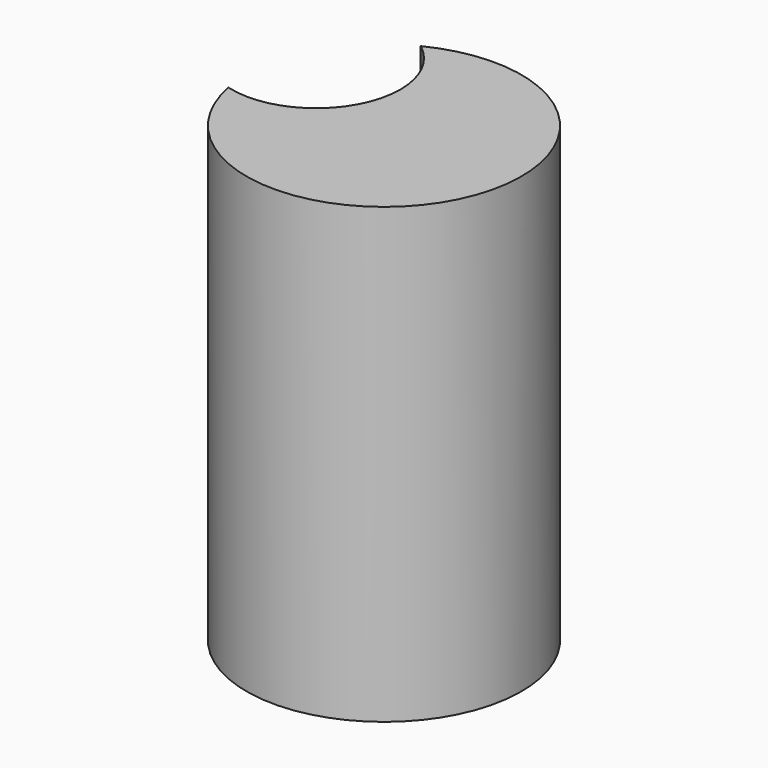
from build123d import *

# Parameters (mm, degrees)
F4_DEPTH = 250.7833242416


# Not quite as in the source:
# - the program builds the solid bodies; features that only make, move or delete a surface that nothing else refers to are left out


with BuildPart() as f4:
    # F3 (on Top) → F4 (new body)
    with BuildSketch(Plane.XY):
        with BuildLine():
            ThreePointArc((109.6018990825, 37.208231044), (123.2300037406, 20.7793931517), (128.1135241215, 0))
            ThreePointArc((128.1135241215, 0), (109.6811059838, -37.1481989447), (68.9499571053, -44.9402612059))
            ThreePointArc((68.9499571053, -44.9402612059), (150.7816116965, -106.503589559), (219.7245289572, -30.7847857475))
            ThreePointArc((219.7245289572, -30.7847857475), (183.6272508744, 33.9261946633), (109.6018990825, 37.208231044))
        make_face()
    extrude(amount=F4_DEPTH)


solid = f4.part
